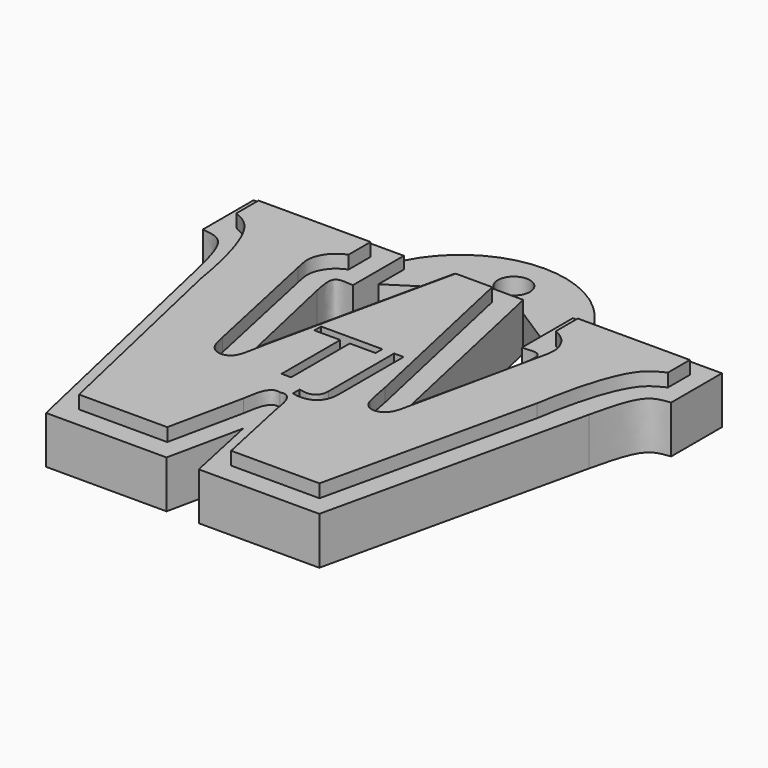
from build123d import *

# Parameters (mm, degrees)
F1_DEPTH     = 6
F2_DEPTH     = 4.7
F0_R         = 1.5875
F3_DEPTH     = 3.5
F4_TEXT_SIZE = 11.336351112
F5_DEPTH     = 25


# Not quite as in the source:
# - Text() gives the source's letters only with a copy of the font that has no kerning and outlines rounded to 1/6400 em; it was checked with that copy


with BuildPart() as f1:
    # F0 (on Top) → F1 (new body)
    with BuildSketch(Plane.XY):
        with BuildLine():
            Line((-10.7832718641, 17.2090474516), (-21.8836143613, 17.2090474516))
            Line((-21.8836143613, 17.2090474516), (-21.8836143613, 14.5007176325))
            add(Edge.make_bspline(
                [(-21.8836143613, 14.5007176325), (-21.2611631485, 14.2003330034), (-19.7222853742, 13.4576961189), (-17.9879653323, 8.7695463348), (-17.4579131706, 5.7032101265), (-17.1917192638, 4.163286183)],
                knots=[0, 0, 0, 0, 0.2526780268, 0.6246924923, 1, 1, 1, 1], degree=3))
            Line((-17.1917192638, 4.163286183), (-12.4295783581, -16.8267668236))
            Line((-12.4295783581, -16.8267668236), (-3.6882117856, -16.8267668236))
            Line((-3.6882117856, -16.8267668236), (-2.1041406426, -9.3932800417))
            add(Edge.make_bspline(
                [(-2.1041406426, -9.3932800417), (-1.9887059101, -8.6368055877), (-1.8008232686, -7.4055607494), (-1.1039871084, -6.7315831446), (-0.7036878821, -6.7944667614), (-0.5244749974, -6.8226195872)],
                knots=[0, 0, 0, 0, 0.4680880514, 0.7618644543, 1, 1, 1, 1], degree=3))
            add(Edge.make_bspline(
                [(1.0551906479, -9.3932800417), (0.9397559153, -8.6368055877), (0.7518732738, -7.4055607494), (0.0550371137, -6.7315831446), (-0.3452621127, -6.7944667614), (-0.5244749974, -6.8226195872)],
                knots=[0, 0, 0, 0, 0.4680880514, 0.7618644543, 1, 1, 1, 1], degree=3))
            Line((1.0551906479, -9.3932800417), (2.6392617909, -16.8267668236))
            Line((2.6392617909, -16.8267668236), (11.3806283634, -16.8267668236))
            Line((11.3806283634, -16.8267668236), (16.142769269, 4.163286183))
            add(Edge.make_bspline(
                [(20.8346643665, 14.5007176325), (20.2122131537, 14.2003330034), (18.6733353794, 13.4576961189), (16.9390153375, 8.7695463348), (16.4089631759, 5.7032101265), (16.142769269, 4.163286183)],
                knots=[0, 0, 0, 0, 0.2526780268, 0.6246924923, 1, 1, 1, 1], degree=3))
            Line((20.8346643665, 14.5007176325), (20.8346643665, 17.2090474516))
            Line((20.8346643665, 17.2090474516), (9.7343218693, 17.2090474516))
            Line((9.7343218693, 17.2090474516), (9.7343218693, 14.5007176325))
            add(Edge.make_bspline(
                [(9.7343218693, 14.5007176325), (10.1021901481, 14.3195963823), (10.9049904537, 13.9243348079), (11.8917716046, 12.246214674), (11.5992273019, 11.0086092041), (11.4508741715, 10.3810029104)],
                knots=[0, 0, 0, 0, 0.2942272373, 0.6420931884, 1, 1, 1, 1], degree=3))
            Line((11.4508741715, 10.3810029104), (8.7043973797, -2.3977414239))
            add(Edge.make_bspline(
                [(8.7043973797, -2.3977414239), (8.5717328494, -3.066290888), (8.3334475195, -4.2671056744), (7.0285853053, -4.8199606382), (5.9416910433, -4.2748030291), (5.6362235784, -2.8471872063), (5.4233856872, -1.7097145764), (5.3094476641, -1.1007939465)],
                knots=[0, 0, 0, 0, 0.2277871211, 0.409139724, 0.5782163911, 0.7742075421, 1, 1, 1, 1], degree=3))
            Line((5.3094476641, -1.1007939465), (1.2812826798, 17.1787862727))
            Line((1.2812826798, 17.1787862727), (-0.5244749974, 17.1787862727))
            Line((-0.5244749974, 17.1787862727), (-2.3302326746, 17.1787862727))
            Line((-2.3302326746, 17.1787862727), (-6.3583976589, -1.1007939465))
            add(Edge.make_bspline(
                [(-9.7533473745, -2.3977414239), (-9.6206828442, -3.066290888), (-9.3823975143, -4.2671056744), (-8.0775353001, -4.8199606382), (-6.9906410381, -4.2748030291), (-6.6851735732, -2.8471872063), (-6.472335682, -1.7097145764), (-6.3583976589, -1.1007939465)],
                knots=[0, 0, 0, 0, 0.2277871211, 0.409139724, 0.5782163911, 0.7742075421, 1, 1, 1, 1], degree=3))
            Line((-9.7533473745, -2.3977414239), (-12.4998241663, 10.3810029104))
            add(Edge.make_bspline(
                [(-10.7832718641, 14.5007176325), (-11.1511401429, 14.3195963823), (-11.9539404484, 13.9243348079), (-12.9407215994, 12.246214674), (-12.6481772966, 11.0086092041), (-12.4998241663, 10.3810029104)],
                knots=[0, 0, 0, 0, 0.2942272373, 0.6420931884, 1, 1, 1, 1], degree=3))
            Line((-10.7832718641, 14.5007176325), (-10.7832718641, 17.2090474516))
        make_face()
    extrude(amount=F1_DEPTH)

    # F0 (on Top) → F2 (join)
    with BuildSketch(Plane.XY):
        with BuildLine():
            Line((22.6048380136, 12.6839569528), (22.6048380136, 18.9609862864))
            Line((22.6048380136, 18.9609862864), (9.2805062269, 18.9609862864))
            Line((9.2805062269, 18.9609862864), (7.8406729915, 18.9609862864))
            Line((7.8406729915, 18.9609862864), (7.8406729915, 15.8062414266))
            Line((7.8406729915, 15.8062414266), (7.8406729915, 12.6514965668))
            add(Edge.make_bspline(
                [(7.8406729915, 12.6514965668), (8.4034247649, 12.7122465313), (9.3318732927, 12.8124740521), (9.8386101583, 12.1387229451), (9.6072547767, 10.971589944), (9.4590499246, 10.2239316329)],
                knots=[0, 0, 0, 0, 0.3561145881, 0.5875309162, 1, 1, 1, 1], degree=3))
            Line((9.4590499246, 10.2239316329), (7.1393768483, -0.1336791611))
            Line((7.1393768483, -0.1336791611), (2.9315962636, 18.9609862864))
            Line((2.9315962636, 18.9609862864), (-0.5244749974, 18.9609862864))
            Line((-0.5244749974, 18.9609862864), (-3.9805462584, 18.9609862864))
            Line((-3.9805462584, 18.9609862864), (-8.1883268431, -0.1336791611))
            Line((-8.1883268431, -0.1336791611), (-10.5079999194, 10.2239316329))
            add(Edge.make_bspline(
                [(-8.8896229863, 12.6514965668), (-9.4523747597, 12.7122465313), (-10.3808232875, 12.8124740521), (-10.887560153, 12.1387229451), (-10.6562047715, 10.971589944), (-10.5079999194, 10.2239316329)],
                knots=[0, 0, 0, 0, 0.3561145881, 0.5875309162, 1, 1, 1, 1], degree=3))
            Line((-8.8896229863, 12.6514965668), (-8.8896229863, 15.8062414266))
            Line((-8.8896229863, 15.8062414266), (-8.8896229863, 18.9609862864))
            Line((-8.8896229863, 18.9609862864), (-10.3294562217, 18.9609862864))
            Line((-10.3294562217, 18.9609862864), (-23.7780641764, 18.9609862864))
            Line((-23.7780641764, 18.9609862864), (-23.7780641764, 12.6989018172))
            add(Edge.make_bspline(
                [(-23.7780641764, 12.6989018172), (-23.1818905633, 12.6275477254), (-21.9765154596, 12.4832802773), (-20.8326476227, 10.8412422697), (-20.2783294273, 8.5113795114), (-19.9471190572, 7.1192644536)],
                knots=[0, 0, 0, 0, 0.282579776, 0.5713346235, 1, 1, 1, 1], degree=3))
            Line((-19.9471190572, 7.1192644536), (-14.0499416739, -18.873680383))
            Line((-14.0499416739, -18.873680383), (-2.1194978617, -18.873680383))
            Line((-2.1194978617, -18.873680383), (-0.5244749974, -11.3888010383))
            Line((-0.5244749974, -11.3888010383), (1.0705478669, -18.873680383))
            Line((1.0705478669, -18.873680383), (13.0009916791, -18.873680383))
            Line((13.0009916791, -18.873680383), (18.8981690624, 7.1192644536))
            add(Edge.make_bspline(
                [(22.6048380136, 12.6839569528), (22.0507118252, 12.6166896187), (20.905097218, 12.4510267999), (19.7836976279, 10.8412422697), (19.2293794325, 8.5113795114), (18.8981690624, 7.1192644536)],
                knots=[0.0196423452, 0.0196423452, 0.0196423452, 0.0196423452, 0.282579776, 0.5713346235, 1, 1, 1, 1], degree=3))
        make_face()
        with BuildLine():
            Line((-21.8836143613, 14.5007176325), (-21.8836143613, 17.2090474516))
            Line((-21.8836143613, 17.2090474516), (-10.7832718641, 17.2090474516))
            Line((-10.7832718641, 17.2090474516), (-10.7832718641, 14.5007176325))
            add(Edge.make_bspline(
                [(-10.7832718641, 14.5007176325), (-11.1511401429, 14.3195963823), (-11.9539404484, 13.9243348079), (-12.9407215994, 12.246214674), (-12.6481772966, 11.0086092041), (-12.4998241663, 10.3810029104)],
                knots=[0, 0, 0, 0, 0.2942272373, 0.6420931884, 1, 1, 1, 1], degree=3))
            Line((-12.4998241663, 10.3810029104), (-9.7533473745, -2.3977414239))
            add(Edge.make_bspline(
                [(-9.7533473745, -2.3977414239), (-9.6206828442, -3.066290888), (-9.3823975143, -4.2671056744), (-8.0775353001, -4.8199606382), (-6.9906410381, -4.2748030291), (-6.6851735732, -2.8471872063), (-6.472335682, -1.7097145764), (-6.3583976589, -1.1007939465)],
                knots=[0, 0, 0, 0, 0.2277871211, 0.409139724, 0.5782163911, 0.7742075421, 1, 1, 1, 1], degree=3))
            Line((-6.3583976589, -1.1007939465), (-2.3302326746, 17.1787862727))
            Line((-2.3302326746, 17.1787862727), (-0.5244749974, 17.1787862727))
            Line((-0.5244749974, 17.1787862727), (1.2812826798, 17.1787862727))
            Line((1.2812826798, 17.1787862727), (5.3094476641, -1.1007939465))
            add(Edge.make_bspline(
                [(8.7043973797, -2.3977414239), (8.5717328494, -3.066290888), (8.3334475195, -4.2671056744), (7.0285853053, -4.8199606382), (5.9416910433, -4.2748030291), (5.6362235784, -2.8471872063), (5.4233856872, -1.7097145764), (5.3094476641, -1.1007939465)],
                knots=[0, 0, 0, 0, 0.2277871211, 0.409139724, 0.5782163911, 0.7742075421, 1, 1, 1, 1], degree=3))
            Line((8.7043973797, -2.3977414239), (11.4508741715, 10.3810029104))
            add(Edge.make_bspline(
                [(9.7343218693, 14.5007176325), (10.1021901481, 14.3195963823), (10.9049904537, 13.9243348079), (11.8917716046, 12.246214674), (11.5992273019, 11.0086092041), (11.4508741715, 10.3810029104)],
                knots=[0, 0, 0, 0, 0.2942272373, 0.6420931884, 1, 1, 1, 1], degree=3))
            Line((9.7343218693, 14.5007176325), (9.7343218693, 17.2090474516))
            Line((9.7343218693, 17.2090474516), (20.8346643665, 17.2090474516))
            Line((20.8346643665, 17.2090474516), (20.8346643665, 14.5007176325))
            add(Edge.make_bspline(
                [(20.8346643665, 14.5007176325), (20.2122131537, 14.2003330034), (18.6733353794, 13.4576961189), (16.9390153375, 8.7695463348), (16.4089631759, 5.7032101265), (16.142769269, 4.163286183)],
                knots=[0, 0, 0, 0, 0.2526780268, 0.6246924923, 1, 1, 1, 1], degree=3))
            Line((16.142769269, 4.163286183), (11.3806283634, -16.8267668236))
            Line((11.3806283634, -16.8267668236), (2.6392617909, -16.8267668236))
            Line((2.6392617909, -16.8267668236), (1.0551906479, -9.3932800417))
            add(Edge.make_bspline(
                [(1.0551906479, -9.3932800417), (0.9397559153, -8.6368055877), (0.7518732738, -7.4055607494), (0.0550371137, -6.7315831446), (-0.3452621127, -6.7944667614), (-0.5244749974, -6.8226195872)],
                knots=[0, 0, 0, 0, 0.4680880514, 0.7618644543, 1, 1, 1, 1], degree=3))
            add(Edge.make_bspline(
                [(-2.1041406426, -9.3932800417), (-1.9887059101, -8.6368055877), (-1.8008232686, -7.4055607494), (-1.1039871084, -6.7315831446), (-0.7036878821, -6.7944667614), (-0.5244749974, -6.8226195872)],
                knots=[0, 0, 0, 0, 0.4680880514, 0.7618644543, 1, 1, 1, 1], degree=3))
            Line((-2.1041406426, -9.3932800417), (-3.6882117856, -16.8267668236))
            Line((-3.6882117856, -16.8267668236), (-12.4295783581, -16.8267668236))
            Line((-12.4295783581, -16.8267668236), (-17.1917192638, 4.163286183))
            add(Edge.make_bspline(
                [(-21.8836143613, 14.5007176325), (-21.2611631485, 14.2003330034), (-19.7222853742, 13.4576961189), (-17.9879653323, 8.7695463348), (-17.4579131706, 5.7032101265), (-17.1917192638, 4.163286183)],
                knots=[0, 0, 0, 0, 0.2526780268, 0.6246924923, 1, 1, 1, 1], degree=3))
        make_face(mode=Mode.SUBTRACT)
    extrude(amount=F2_DEPTH)

    # F0 (on Top) → F3 (join)
    with BuildSketch(Plane.XY):
        with BuildLine():
            Line((7.8406729915, 18.9609862864), (9.2805062269, 18.9609862864))
            ThreePointArc((9.2805062269, 18.9609862864), (-0.5244749974, 25.8888191764), (-10.3294562217, 18.9609862864))
            Line((-10.3294562217, 18.9609862864), (-8.8896229863, 18.9609862864))
            Line((-8.8896229863, 18.9609862864), (-8.8896229863, 15.8062414266))
            Line((-8.8896229863, 15.8062414266), (-3.9805462584, 18.9609862864))
            Line((-3.9805462584, 18.9609862864), (-0.5244749974, 18.9609862864))
            Line((-0.5244749974, 18.9609862864), (2.9315962636, 18.9609862864))
            Line((2.9315962636, 18.9609862864), (7.8406729915, 15.8062414266))
            Line((7.8406729915, 15.8062414266), (7.8406729915, 18.9609862864))
        make_face()
        with Locations((-0.5244749974, 22.1202913672)):
            Circle(F0_R, mode=Mode.SUBTRACT)
    extrude(amount=F3_DEPTH)

    # F4 (on face) → F5 (cut)
    with BuildSketch(Plane.XY.offset(6)):
        with Locations((-5.0247575466, -4.3286996051)):
            Text('TJ', F4_TEXT_SIZE, font='Open Sans', text_align=(TextAlign.LEFT, TextAlign.BOTTOM))
    extrude(amount=-F5_DEPTH, mode=Mode.SUBTRACT)


solid = f1.part
